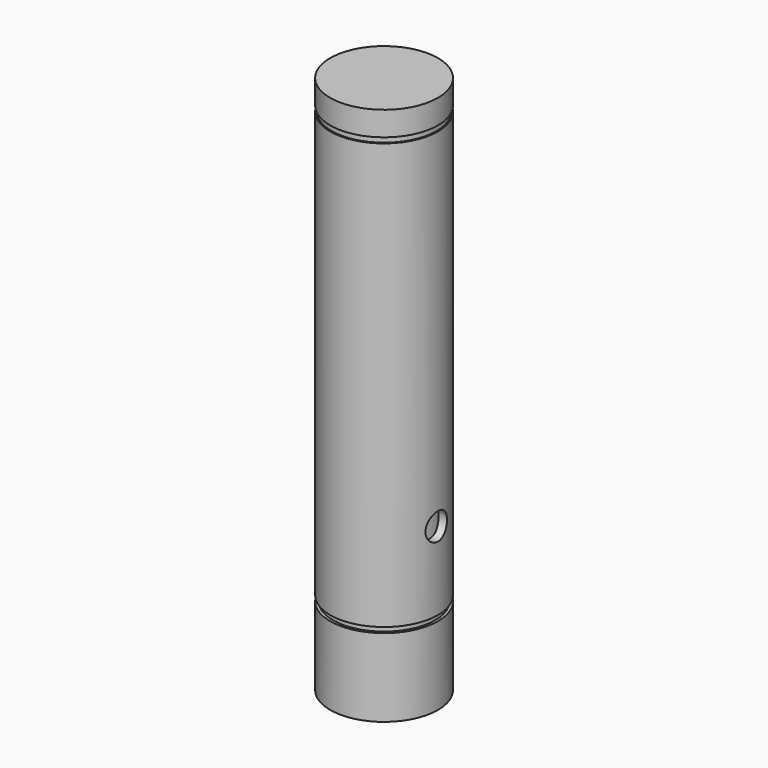
from build123d import *

# Parameters (mm, degrees)
F0_R      = 10
F0_R_2    = 8.5
F1_DEPTH  = 50
F2_R      = 8.5
F3_DEPTH  = 1.5
F4_R      = 2.5
F5_DEPTH  = 12.5
F7_R      = 10
F7_R_2    = 9.75
F8_DEPTH  = 0.5
F10_R     = 10
F10_R_2   = 9.5
F11_DEPTH = 0.5


# Not quite as in the source:
# - a pattern or mirror of a feature is missing from the dataset's text; its kind, count and spacing are read off the source's solid


with BuildPart() as f1:
    # F0 (on Top) → F1 (new body, symmetric)
    with BuildSketch(Plane.XY):
        Circle(F0_R)
        Circle(F0_R_2, mode=Mode.SUBTRACT)
    extrude(amount=F1_DEPTH, both=True)

    # F2 (on face) → F3 (join)
    with BuildSketch(Plane.XY.offset(50)):
        Circle(F2_R)
    f3 = extrude(amount=-F3_DEPTH)

    # F3_copies: F3 across plane
    add(f3.mirror(Plane(origin=(0, 0, 0), x_dir=(-1, 0, 0), z_dir=(0, 0, -1))))

    # F4 (on Right) → F5 (cut, symmetric)
    with BuildSketch(Plane.YZ):
        with Locations((0, -20)):
            Circle(F4_R)
    extrude(amount=F5_DEPTH, both=True, mode=Mode.SUBTRACT)

    # F7 (on offset) → F8 (cut, symmetric)
    with BuildSketch(Plane.XY.offset(45)):
        Circle(F7_R)
        Circle(F7_R_2, mode=Mode.SUBTRACT)
    extrude(amount=F8_DEPTH, both=True, mode=Mode.SUBTRACT)

    # F10 (on face) → F11 (cut, symmetric)
    with BuildSketch(Plane(origin=(0, 0, -35), x_dir=(1, 0, 0), z_dir=(0, 0, -1))):
        Circle(F10_R)
        Circle(F10_R_2, mode=Mode.SUBTRACT)
    extrude(amount=F11_DEPTH, both=True, mode=Mode.SUBTRACT)


solid = f1.part
